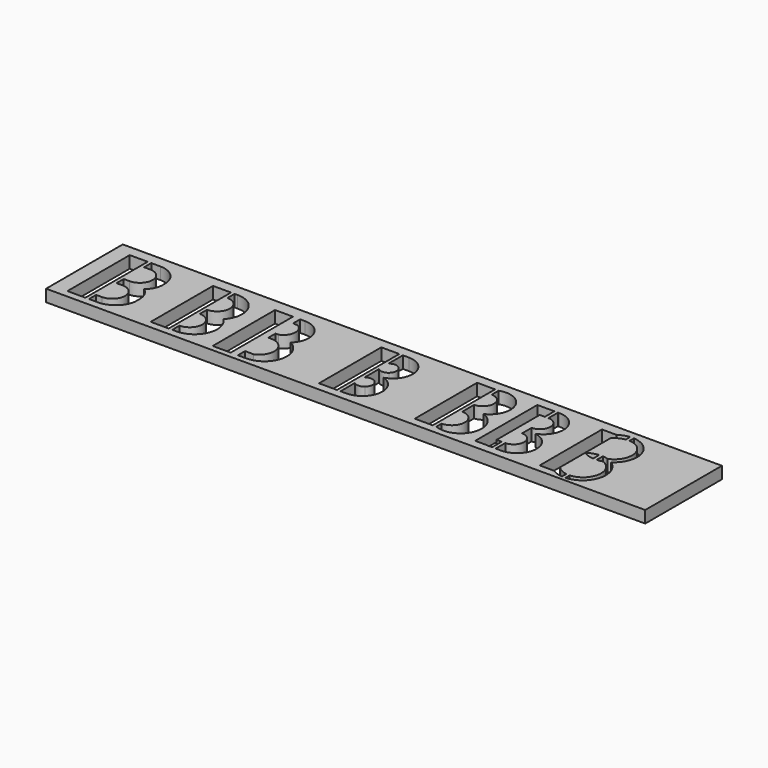
from build123d import *

# Parameters (mm, degrees)
F0_W      = 1270
F0_H      = 203.2
F1_DEPTH  = 25.4
F3_DEPTH  = 25.4
F5_DEPTH  = 25.4
F6_W      = 38.1
F6_H      = 165.1
F7_DEPTH  = 25.4
F8_W      = 38.1
F8_H      = 165.1
F9_DEPTH  = 25.4
F10_W     = 38.1
F10_H     = 165.1
F11_DEPTH = 25.4
F12_W     = 10.8188445342
F12_H     = 25.4
F13_DEPTH = 25.4
F15_DEPTH = 25.4


# Not quite as in the source:
# - a feature names something its author has since deleted; it is built from what else it names


with BuildPart() as f1:
    # F0 (on Top) → F1 (new body)
    with BuildSketch(Plane.XY):
        with Locations((-238.9351708174, -1032.4661802616)):
            Rectangle(F0_W, F0_H)
    extrude(amount=F1_DEPTH)

    # F2 (on face) → F3 (cut)
    with BuildSketch(Plane.XY.offset(25.4)):
        Polygon((-802.8773658486, -953.6430131912), (-840.9773658486, -953.6430131912), (-840.9773658486, -1118.7430131912), (-802.8773658486, -1118.7430131912), (-802.8773658486, -1036.1930131912), align=None)
        with BuildLine():
            Line((-795.2573658486, -1026.6680131912), (-795.2573658486, -1034.9226884847))
            ThreePointArc((-795.2573658486, -1034.9226884847), (-770.7707510059, -1026.0470401418), (-745.9674756926, -1033.9949312892))
            ThreePointArc((-745.9674756926, -1033.9949312892), (-735.9296714012, -1021.4477610393), (-731.4022587776, -1006.0305131912))
            Line((-731.4022587776, -1006.0305131912), (-731.4022587776, -993.3305131912))
            ThreePointArc((-731.4022587776, -993.3305131912), (-746.2799733966, -964.9916145085), (-776.2073658486, -953.6430131912))
            Line((-776.2073658486, -953.6430131912), (-795.2573658486, -953.6430131912))
            Line((-795.2573658486, -953.6430131912), (-795.2573658486, -972.6930131912))
            Line((-795.2573658486, -972.6930131912), (-782.5573658486, -972.6930131912))
            ThreePointArc((-782.5573658486, -972.6930131912), (-755.5698658486, -999.6805131912), (-782.5573658486, -1026.6680131912))
            Line((-782.5573658486, -1026.6680131912), (-795.2573658486, -1026.6680131912))
        make_face()
        with BuildLine():
            ThreePointArc((-745.9674756926, -1033.9949312892), (-770.0833121416, -1043.7192190255), (-795.2573658486, -1037.2075096056))
            Line((-795.2573658486, -1037.2075096056), (-795.2573658486, -1045.7180131912))
            Line((-795.2573658486, -1045.7180131912), (-782.5573658486, -1045.7180131912))
            ThreePointArc((-782.5573658486, -1045.7180131912), (-755.5698658486, -1072.7055131912), (-782.5573658486, -1099.6930131912))
            Line((-782.5573658486, -1099.6930131912), (-795.2573658486, -1099.6930131912))
            Line((-795.2573658486, -1099.6930131912), (-795.2573658486, -1118.7430131912))
            Line((-795.2573658486, -1118.7430131912), (-776.2073658486, -1118.7430131912))
            ThreePointArc((-776.2073658486, -1118.7430131912), (-745.6362827432, -1107.4726468348), (-729.6964334488, -1079.0555131912))
            Line((-729.6964334488, -1079.0555131912), (-729.6964334488, -1066.3555131912))
            ThreePointArc((-729.6964334488, -1066.3555131912), (-733.9931607032, -1048.2450598787), (-745.9674756926, -1033.9949312892))
        make_face()
        with BuildLine():
            Line((-795.2573658486, -1034.9226884847), (-795.2573658486, -1036.1930131912))
            Line((-795.2573658486, -1036.1930131912), (-795.2573658486, -1037.2075096056))
            ThreePointArc((-795.2573658486, -1037.2075096056), (-770.0833121416, -1043.7192190255), (-745.9674756926, -1033.9949312892))
            ThreePointArc((-745.9674756926, -1033.9949312892), (-770.7707510059, -1026.0470401418), (-795.2573658486, -1034.9226884847))
        make_face()
    extrude(amount=-F3_DEPTH, mode=Mode.SUBTRACT)

    # F4 (on face) → F5 (cut)
    with BuildSketch(Plane.XY.offset(25.4)):
        Polygon((-626.2925520338, -953.6430131912), (-664.3925520338, -953.6430131912), (-664.3925520338, -1118.7430131912), (-626.2925520338, -1118.7430131912), (-626.2925520338, -1036.1930131912), align=None)
        with BuildLine():
            Line((-618.6725520338, -1026.6680131912), (-618.6725520338, -1036.1930131912))
            Line((-618.6725520338, -1036.1930131912), (-576.4699598814, -1036.1930131912))
            ThreePointArc((-576.4699598814, -1036.1930131912), (-567.2333827461, -983.181698655), (-612.2109314466, -953.6430131912))
            Line((-612.2109314466, -953.6430131912), (-618.6725520338, -953.6430131912))
            Line((-618.6725520338, -953.6430131912), (-618.6725520338, -972.6930131912))
            ThreePointArc((-618.6725520338, -972.6930131912), (-591.6850520338, -999.6805131912), (-618.6725520338, -1026.6680131912))
        make_face()
        with BuildLine():
            Line((-576.4699598814, -1036.1930131912), (-618.6725520338, -1036.1930131912))
            Line((-618.6725520338, -1036.1930131912), (-618.6725520338, -1045.7180131912))
            ThreePointArc((-618.6725520338, -1045.7180131912), (-591.6850520338, -1072.7055131912), (-618.6725520338, -1099.6930131912))
            Line((-618.6725520338, -1099.6930131912), (-618.6725520338, -1118.7430131912))
            Line((-618.6725520338, -1118.7430131912), (-609.5818281174, -1118.7430131912))
            ThreePointArc((-609.5818281174, -1118.7430131912), (-565.110212681, -1088.6653525193), (-576.4699598814, -1036.1930131912))
        make_face()
    extrude(amount=-F5_DEPTH, mode=Mode.SUBTRACT)

    # F6 (on face) → F7 (cut)
    with BuildSketch(Plane.XY.offset(25.4)):
        with Locations((-290.2511896121, -1034.2057645321)):
            Rectangle(F6_W, F6_H)
        with BuildLine():
            Line((-250.8811896121, -951.6557645321), (-263.5811896121, -951.6557645321))
            Line((-263.5811896121, -951.6557645321), (-263.5811896121, -989.7557645321))
            ThreePointArc((-263.5811896121, -989.7557645321), (-253.0317773062, -985.9457645321), (-242.4823650003, -989.7557645321))
            ThreePointArc((-242.4823650003, -989.7557645321), (-236.5217773062, -1002.4557645321), (-242.4823650003, -1015.1557645321))
            ThreePointArc((-242.4823650003, -1015.1557645321), (-253.0317773062, -1018.9657645321), (-263.5811896121, -1015.1557645321))
            Line((-263.5811896121, -1015.1557645321), (-263.5811896121, -1034.2057645321))
            Line((-263.5811896121, -1034.2057645321), (-238.1811896121, -1034.2057645321))
            ThreePointArc((-238.1811896121, -1034.2057645321), (-209.1205846715, -987.4829791566), (-250.8811896121, -951.6557645321))
        make_face()
        with BuildLine():
            ThreePointArc((-250.8811896121, -1116.7557645321), (-209.1205846715, -1080.9285499076), (-238.1811896121, -1034.2057645321))
            Line((-238.1811896121, -1034.2057645321), (-263.5811896121, -1034.2057645321))
            Line((-263.5811896121, -1034.2057645321), (-263.5811896121, -1053.2557645321))
            ThreePointArc((-263.5811896121, -1053.2557645321), (-253.0317773062, -1049.4457645321), (-242.4823650003, -1053.2557645321))
            ThreePointArc((-242.4823650003, -1053.2557645321), (-236.5217773062, -1065.9557645321), (-242.4823650003, -1078.6557645321))
            ThreePointArc((-242.4823650003, -1078.6557645321), (-253.0317773062, -1082.4657645321), (-263.5811896121, -1078.6557645321))
            Line((-263.5811896121, -1078.6557645321), (-263.5811896121, -1116.7557645321))
            Line((-263.5811896121, -1116.7557645321), (-250.8811896121, -1116.7557645321))
        make_face()
    extrude(amount=-F7_DEPTH, mode=Mode.SUBTRACT)

    # F8 (on face) → F9 (cut)
    with BuildSketch(Plane.XY.offset(25.4)):
        with Locations((-511.1800421023, -1039.6600419521)):
            Rectangle(F8_W, F8_H)
        with BuildLine():
            Line((-476.8900421023, -1103.1600419521), (-476.8900421023, -1122.2100419521))
            Line((-476.8900421023, -1122.2100419521), (-458.6642896088, -1122.2100419521))
            ThreePointArc((-458.6642896088, -1122.2100419521), (-412.3120735256, -1085.6240501252), (-437.1304200925, -1032.0412879019))
            ThreePointArc((-437.1304200925, -1032.0412879019), (-426.7974991694, -984.4173911629), (-467.1597770349, -957.1100419521))
            Line((-467.1597770349, -957.1100419521), (-476.8900421023, -957.1100419521))
            Line((-476.8900421023, -957.1100419521), (-476.8900421023, -976.1600419521))
            Line((-476.8900421023, -976.1600419521), (-467.1597770349, -976.1600419521))
            ThreePointArc((-467.1597770349, -976.1600419521), (-453.8301047521, -1000.5208961567), (-470.7810375499, -1022.5162879019))
            Line((-470.7810375499, -1022.5162879019), (-476.8900421023, -1022.5162879019))
            Line((-476.8900421023, -1022.5162879019), (-476.8900421023, -1041.5662879019))
            Line((-476.8900421023, -1041.5662879019), (-470.7810375499, -1041.5662879019))
            ThreePointArc((-470.7810375499, -1041.5662879019), (-439.3939139214, -1067.38048316), (-458.6642896088, -1103.1600419521))
            Line((-458.6642896088, -1103.1600419521), (-476.8900421023, -1103.1600419521))
        make_face()
    extrude(amount=-F9_DEPTH, mode=Mode.SUBTRACT)

    # F10 (on face) → F11 (cut)
    with BuildSketch(Plane.XY.offset(25.4)):
        with BuildLine():
            ThreePointArc((-28.1148758721, -1032.6774345846), (-5.6831499313, -976.6978639922), (-60.5446838784, -951.6557645321))
            Line((-60.5446838784, -951.6557645321), (-60.5446838784, -970.1407297723))
            ThreePointArc((-60.5446838784, -970.1407297723), (-37.3573787729, -993.3280348778), (-60.5446838784, -1016.5153399833))
            Line((-60.5446838784, -1016.5153399833), (-60.5446838784, -1048.1804596051))
            ThreePointArc((-60.5446838784, -1048.1804596051), (-33.2443789514, -1075.4807645321), (-60.5446838784, -1102.7810694591))
            Line((-60.5446838784, -1102.7810694591), (-60.5446838784, -1116.7557645321))
            ThreePointArc((-60.5446838784, -1116.7557645321), (-0.2627634404, -1091.713665072), (-28.1148758721, -1032.6774345846))
        make_face()
        with Locations((-87.2146838784, -1034.2057645321)):
            Rectangle(F10_W, F10_H)
    extrude(amount=-F11_DEPTH, mode=Mode.SUBTRACT)

    # F12 (on face) → F13 (cut)
    with BuildSketch(Plane.XY.offset(25.4)):
        Polygon((46.8103381641, -977.0557645321), (46.8103381641, -951.6557645321), (21.4103381641, -951.6557645321), (21.4103381641, -1116.2804365158), (46.8103381641, -1116.2804365158), (46.8103381641, -1091.3557645321), (46.8103381641, -1046.9057645321), (46.8103381641, -1034.2057645321), (46.8103381641, -1021.5057645321), align=None)
        with Locations((52.2197604311, -964.3557645321)):
            Rectangle(F12_W, F12_H)
        Polygon((46.8103381641, -1091.3557645321), (46.8103381641, -1116.2804365158), (46.8103381641, -1116.7557645321), (57.6291826982, -1116.7557645321), (57.6291826982, -1091.3557645321), align=None)
        with BuildLine():
            ThreePointArc((65.2491826982, -977.0557645321), (87.4741826982, -999.2807645321), (65.2491826982, -1021.5057645321))
            Line((65.2491826982, -1021.5057645321), (65.2491826982, -1034.2057645321))
            Line((65.2491826982, -1034.2057645321), (83.540642596, -1034.2057645321))
            ThreePointArc((83.540642596, -1034.2057645321), (110.4072024463, -986.6390604349), (68.4480272324, -951.6557645321))
            Line((68.4480272324, -951.6557645321), (65.2491826982, -951.6557645321))
            Line((65.2491826982, -951.6557645321), (65.2491826982, -977.0557645321))
        make_face()
        with BuildLine():
            Line((83.540642596, -1034.2057645321), (65.2491826982, -1034.2057645321))
            Line((65.2491826982, -1034.2057645321), (65.2491826982, -1046.9057645321))
            ThreePointArc((65.2491826982, -1046.9057645321), (87.4741826982, -1069.1307645321), (65.2491826982, -1091.3557645321))
            Line((65.2491826982, -1091.3557645321), (65.2491826982, -1116.7557645321))
            Line((65.2491826982, -1116.7557645321), (77.190642596, -1116.7557645321))
            ThreePointArc((77.190642596, -1116.7557645321), (118.587577869, -1078.4209133992), (83.540642596, -1034.2057645321))
        make_face()
    extrude(amount=-F13_DEPTH, mode=Mode.SUBTRACT)

    # F14 (on face) → F15 (cut)
    with BuildSketch(Plane.XY.offset(25.4)):
        with BuildLine():
            Line((213.370859623, -1126.6048977295), (213.370859623, -1114.9853357906))
            ThreePointArc((213.370859623, -1114.9853357906), (200.773188913, -1110.8213233384), (190.3673261404, -1102.5897787094))
            Line((190.3673261404, -1102.5897787094), (190.3673261404, -969.2397787094))
            ThreePointArc((190.3673261404, -969.2397787094), (200.7161524236, -961.0863132759), (213.2232278912, -956.9450251593))
            Line((213.2232278912, -956.9450251593), (212.9195398237, -945.3366661787))
            ThreePointArc((212.9195398237, -945.3366661787), (201.1512347814, -947.9680613325), (190.3673261404, -953.3647787094))
            Line((190.3673261404, -953.3647787094), (159.8152369261, -953.3647787094))
            Line((159.8152369261, -953.3647787094), (159.8152369261, -1118.3487176895))
            Line((159.8152369261, -1118.3487176895), (190.3673261404, -1118.4647787094))
            ThreePointArc((190.3673261404, -1118.4647787094), (201.3599627311, -1123.9736123253), (213.370859623, -1126.6048977295))
        make_face()
        with BuildLine():
            ThreePointArc((233.0341281328, -1029.9670075356), (227.08706533, -1028.3938294356), (220.990859623, -1027.569984006))
            Line((220.990859623, -1027.569984006), (220.990859623, -1044.0753467383))
            ThreePointArc((220.990859623, -1044.0753467383), (226.9749905665, -1043.3169006739), (232.8225876525, -1041.8368088181))
            ThreePointArc((232.8225876525, -1041.8368088181), (256.4621416526, -1083.337416125), (220.990859623, -1115.3204908886))
            Line((220.990859623, -1115.3204908886), (220.990859623, -1126.7132278679))
            ThreePointArc((220.990859623, -1126.7132278679), (265.7478847903, -1090.0150099575), (245.143692557, -1035.9278787521))
            ThreePointArc((245.143692557, -1035.9278787521), (265.6385890404, -981.8947740671), (220.990859623, -945.2042106805))
            Line((220.990859623, -945.2042106805), (220.990859623, -956.6048305363))
            ThreePointArc((220.990859623, -956.6048305363), (256.3621577318, -988.4678247955), (233.0341281328, -1029.9670075356))
        make_face()
        with BuildLine():
            Line((191.6592419147, -1035.0634215308), (191.6592419147, -1036.7437991805))
            ThreePointArc((191.6592419147, -1036.7437991805), (202.0911371494, -1041.6354927603), (213.370859623, -1043.9851661811))
            Line((213.370859623, -1043.9851661811), (213.370859623, -1027.6066599284))
            ThreePointArc((213.370859623, -1027.6066599284), (202.0728981967, -1030.0476390226), (191.6592419147, -1035.0634215308))
        make_face()
    extrude(amount=-F15_DEPTH, mode=Mode.SUBTRACT)


solid = f1.part
